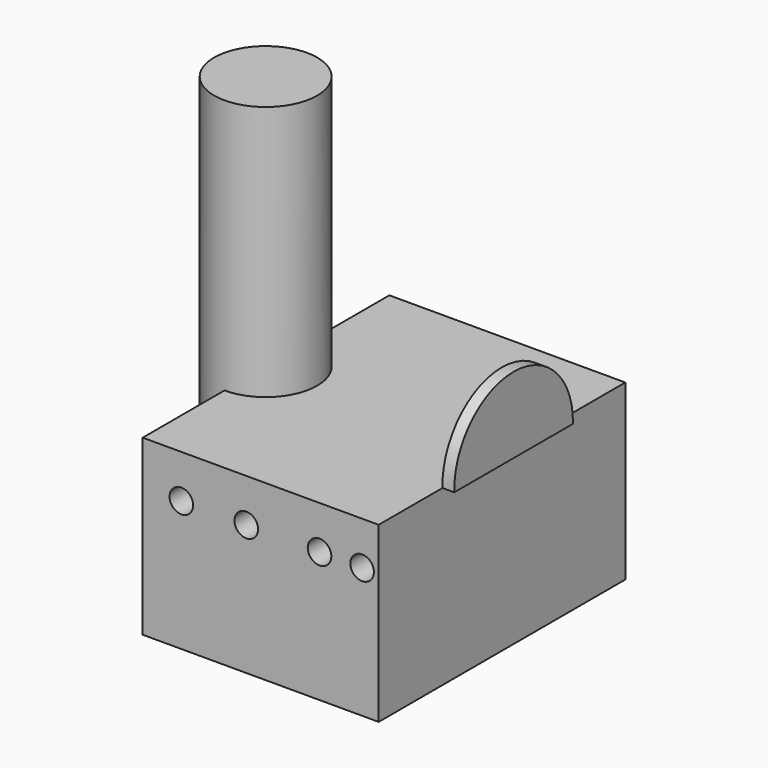
from build123d import *

# Parameters (mm, degrees)
F0_R     = 110.9807708896
F1_DEPTH = 736.6
F2_W     = 663.6773943901
F2_H     = 373.6258000135
F3_DEPTH = 508
F5_DEPTH = 25.4
F7_DEPTH = 25.4
F9_DEPTH = 162.56
F11_D    = 50.8


with BuildPart() as f1:
    # F0 (on Top) → F1 (new body)
    with BuildSketch(Plane.XY):
        Circle(F0_R)
    extrude(amount=F1_DEPTH)

    # F2 (on Right) → F3 (join)
    with BuildSketch(Plane.YZ):
        with Locations((0.9217560291, -0.1024082303)):
            Rectangle(F2_W, F2_H)
    extrude(amount=F3_DEPTH)

    # F6 (on face) → F7 (join)
    with BuildSketch(Plane(origin=(0, 0, 0), x_dir=(1, 0, 0), z_dir=(0, 0, -1))):
        with BuildLine():
            Line((0, -110.9807708896), (0, 110.9807708896))
            ThreePointArc((0, 110.9807708896), (-110.9807708896, 0), (0, -110.9807708896))
        make_face()
    extrude(amount=F7_DEPTH)

    # F8 (on face) → F9 (join)
    with BuildSketch(Plane(origin=(0, 0, -25.4), x_dir=(1, 0, 0), z_dir=(0, 0, -1))):
        with BuildLine():
            Line((0, -110.9807708896), (0, 110.9807708896))
            ThreePointArc((0, 110.9807708896), (-110.9807708896, 0), (0, -110.9807708896))
        make_face()
    extrude(amount=F9_DEPTH)

    # F11 (through all)
    with Locations(Plane.XZ.offset(330.9169411659)):
        with Locations((83.1505954266, 93.6952754855), (222.9530066252, 93.6952754855), (380.6501328945, 93.6952754855), (472.3605215549, 93.6952754855)):
            Hole(F11_D / 2)


with BuildPart() as f5:
    # F4 (on face) → F5 (new body)
    with BuildSketch(Plane.YZ.offset(508)):
        with BuildLine():
            Line((-159.3900769949, 186.7104917765), (160.1164340973, 186.7104917765))
            ThreePointArc((160.1164340973, 186.7104917765), (0.3631785512, 350.410705947), (-159.3900769949, 186.7104917765))
        make_face()
    extrude(amount=F5_DEPTH)


solid = Compound([f1.part, f5.part])
